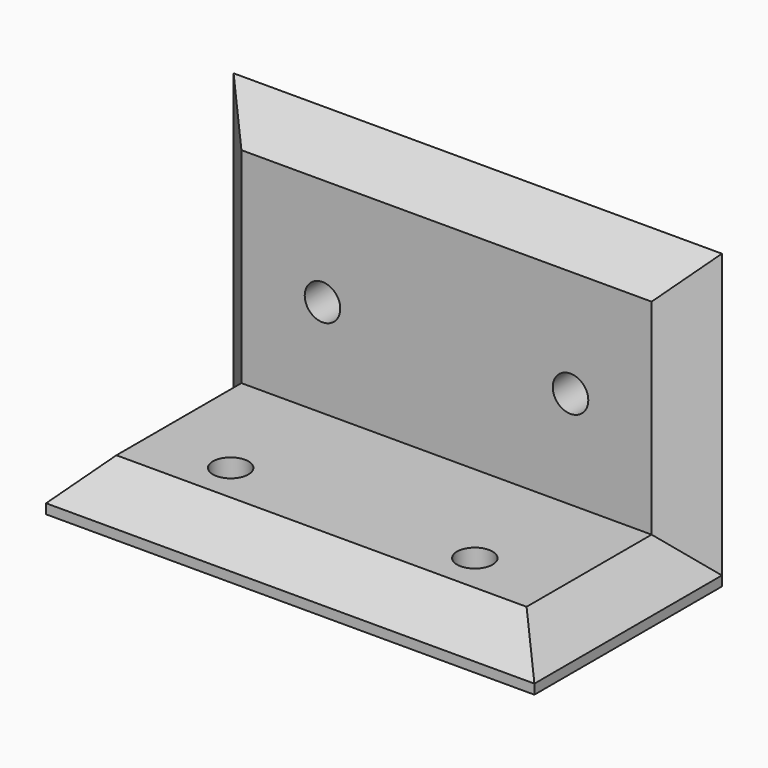
from build123d import *

# Parameters (mm, degrees)
F1_DEPTH = 5.08
F2_W     = 63.5
F2_H     = 6.35
F3_DEPTH = 25.4
F4_R     = 2.3114
F5_DEPTH = 25.4
F6_SIZE  = 5.07999


# Not quite as in the source:
# - a fillet or chamfer is up to 0.001 mm smaller than in the source, because OpenCascade refuses the exact size


with BuildPart() as f1:
    # F0 (on Front) → F1 (new body)
    with BuildSketch(Plane.XZ):
        Polygon((0, 19.05), (0, 0), (31.75, 0), (31.75, 38.1), (30.7521958955, 38.1), (0, 38.1), align=None)
        with BuildLine():
            ThreePointArc((17.9369489739, 19.05), (15.6255489739, 16.7386), (13.3141489739, 19.05))
            ThreePointArc((13.3141489739, 19.05), (15.6255489739, 21.3614), (17.9369489739, 19.05))
        make_face(mode=Mode.SUBTRACT)
        Polygon((31.75, 38.1), (31.75, 0), (63.5, 0), (63.5, 19.05), (63.5, 38.1), (32.7478041045, 38.1), align=None)
        with BuildLine():
            ThreePointArc((45.5630510261, 19.05), (47.8744510261, 21.3614), (50.1858510261, 19.05))
            ThreePointArc((50.1858510261, 19.05), (47.8744510261, 16.7386), (45.5630510261, 19.05))
        make_face(mode=Mode.SUBTRACT)
    extrude(amount=F1_DEPTH)

    # F2 (on face) → F3 (join)
    with BuildSketch(Plane.XZ.offset(5.08)):
        with Locations((31.75, 3.175)):
            Rectangle(F2_W, F2_H)
    extrude(amount=F3_DEPTH)

    # F4 (on face) → F5 (cut)
    with BuildSketch(Plane.XY.offset(6.35)):
        with Locations((15.875, -20.32)):
            Circle(F4_R)
        with Locations((47.625, -20.32)):
            Circle(F4_R)
    extrude(amount=-F5_DEPTH, mode=Mode.SUBTRACT)

    # F6 (size 5.08 in the source; OpenCascade refuses exactly that, so slightly less here)
    f6_edges = [f1.edges().sort_by_distance(p)[0] for p in [
        (31.75, -5.08, 38.1),
        (31.75, -30.48, 6.35),
        (0, -17.78, 6.35),
        (63.5, -17.78, 6.35),
        (0, -5.08, 22.225),
        (63.5, -5.08, 22.225),
    ]]
    chamfer(f6_edges, length=F6_SIZE)


solid = f1.part
